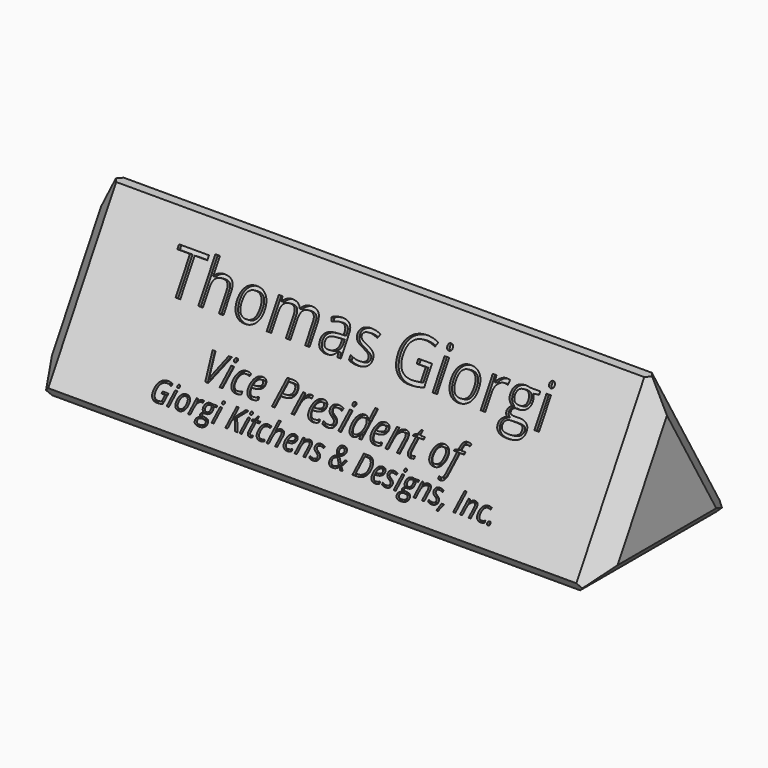
from build123d import *

# Parameters (mm, degrees)
F0_W           = 150
F0_H           = 50
F1_DEPTH       = 100
F3_DEPTH       = 150.001
F4_SIZE        = 5
F5_SIZE        = 2.5
F6_TEXT_SIZE   = 14.894977057
F6_TEXT_SIZE_2 = 9.4105784985
F6_TEXT_SIZE_3 = 6.9444444444
F7_DEPTH       = 1
F8_TEXT_SIZE   = 11.0773833622
F8_TEXT_SIZE_2 = 8.3548943196
F8_TEXT_SIZE_3 = 6.6324197624
F8_TEXT_SIZE_4 = 8.6575247779
F9_DEPTH       = 1


# Not quite as in the source:
# - Text() gives the source's letters only with a copy of the font that has no kerning and outlines rounded to 1/6400 em; it was checked with that copy


with BuildPart() as f1:
    # F0 (on Top) → F1 (new body)
    with BuildSketch(Plane.XY):
        Rectangle(F0_W, F0_H)
    extrude(amount=F1_DEPTH)

    # F2 (on face) → F3 (cut, through all)
    with BuildSketch(Plane.YZ.offset(75)):
        Polygon((-25, 100), (-25, 0), (0, 43.3012701892), (25, 0), (25, 100), align=None)
    extrude(amount=-F3_DEPTH, mode=Mode.SUBTRACT)

    # F4
    f4_edges = [f1.edges().sort_by_distance(p)[0] for p in [
        (75, -12.5, 21.650635),
        (75, 12.5, 21.650635),
        (75, 0, 0),
        (-75, 12.5, 21.650635),
        (-75, -12.5, 21.650635),
        (-75, 0, 0),
    ]]
    chamfer(f4_edges, length=F4_SIZE)

    # F5
    f5_edges = [f1.edges().sort_by_distance(p)[0] for p in [
        (0, 0, 43.30127),
        (0, 25, 0),
        (0, -25, 0),
    ]]
    chamfer(f5_edges, length=F5_SIZE)

    # F6 (on face) → F7 (cut)
    with BuildSketch(Plane(origin=(0, -18.75, 10.8253175473), x_dir=(1, 0, 0), z_dir=(0, -0.8660254038, 0.5))):
        with Locations((-50.4567347807, 16.7756165189)):
            Text('Thomas Giorgi', F6_TEXT_SIZE, font='Open Sans', text_align=(TextAlign.LEFT, TextAlign.BOTTOM))
        with Locations((-35, 2.5)):
            Text('Vice President of', F6_TEXT_SIZE_2, font='Open Sans', font_style=FontStyle.ITALIC, text_align=(TextAlign.LEFT, TextAlign.BOTTOM))
        with Locations((-45.5154079861, -5)):
            Text('Giorgi Kitchens & Designs, Inc.', F6_TEXT_SIZE_3, font='Open Sans', font_style=FontStyle.ITALIC, text_align=(TextAlign.LEFT, TextAlign.BOTTOM))
    extrude(amount=-F7_DEPTH, mode=Mode.SUBTRACT)

    # F8 (on face) → F9 (cut)
    with BuildSketch(Plane(origin=(0, 18.75, 10.8253175473), x_dir=(-1, 0, 0), z_dir=(0, 0.8660254038, 0.5))):
        with Locations((-51.9529279689, 22.0242839792)):
            Text('Giorgi Craftsmanship', F8_TEXT_SIZE, font='Open Sans', font_style=FontStyle.ITALIC, text_align=(TextAlign.LEFT, TextAlign.BOTTOM))
        with Locations((-36.8555275674, 11.0087600691)):
            Text('MADE IN THE USA', F8_TEXT_SIZE_2, font='Open Sans', font_style=FontStyle.BOLD, text_align=(TextAlign.LEFT, TextAlign.BOTTOM))
        with Locations((-36.8555275674, 3.7334178401)):
            Text('Wilmington, Delaware', F8_TEXT_SIZE_3, font='Open Sans', font_style=FontStyle.BOLD, text_align=(TextAlign.LEFT, TextAlign.BOTTOM))
        with Locations((-18.3086357979, -5)):
            Text('Est. 2010', F8_TEXT_SIZE_4, font='Open Sans', font_style=FontStyle.BOLDITALIC, text_align=(TextAlign.LEFT, TextAlign.BOTTOM))
    extrude(amount=-F9_DEPTH, mode=Mode.SUBTRACT)


solid = f1.part
